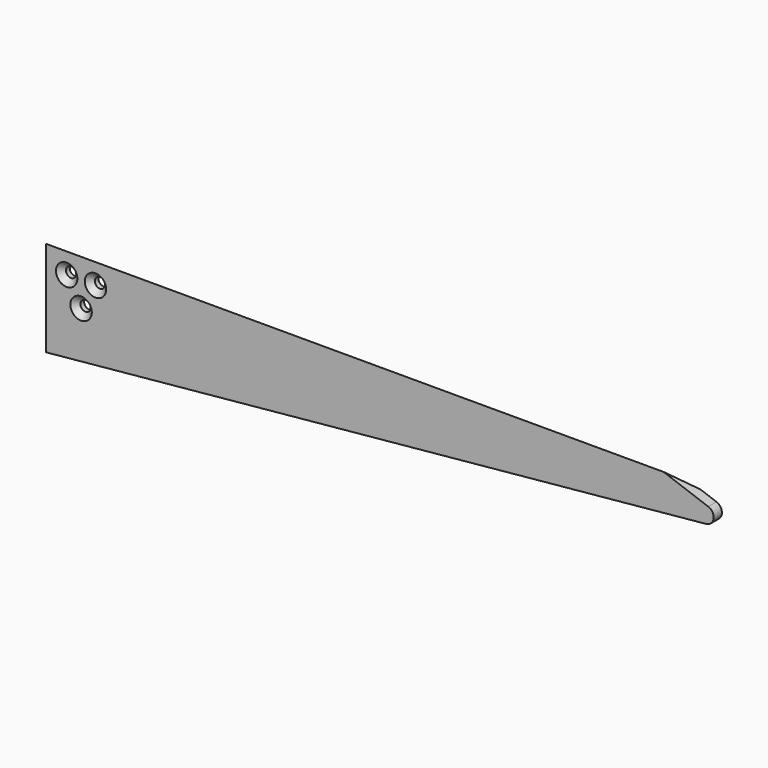
from build123d import *

# Parameters (mm, degrees)
F1_DEPTH       = 6.35
F3_D           = 6.35
F3_CSINK_D     = 13.208
F3_CSINK_ANGLE = 90
F4_SIZE        = 6.34999


# Not quite as in the source:
# - a fillet or chamfer is up to 0.001 mm smaller than in the source, because OpenCascade refuses the exact size


with BuildPart() as f1:
    # F0 (on Front) → F1 (new body)
    with BuildSketch(Plane.XZ):
        with BuildLine():
            Line((381, 0), (0, 0))
            Line((0, 0), (0, -58.9188076556))
            Line((0, -58.9188076556), (407.243362891, -19.705731858))
            ThreePointArc((407.243362891, -19.705731858), (411.7971966033, -15.2795473621), (408.473715423, -9.868171981))
            Line((408.473715423, -9.868171981), (381, 0))
        make_face()
    extrude(amount=F1_DEPTH)

    # F3 (through all)
    with Locations(Plane.XZ.offset(6.35)):
        with Locations((12.7, -12.7), (30.48, -12.7), (21.59, -28.0979316793)):
            CounterSinkHole(F3_D / 2, F3_CSINK_D / 2, counter_sink_angle=F3_CSINK_ANGLE)

    # F4 (size 6.35 in the source; OpenCascade refuses exactly that, so slightly less here)
    f4_edges = [f1.edges().sort_by_distance(p)[0] for p in [
        (190.5, 0, 0),
    ]]
    chamfer(f4_edges, length=F4_SIZE)


solid = f1.part
